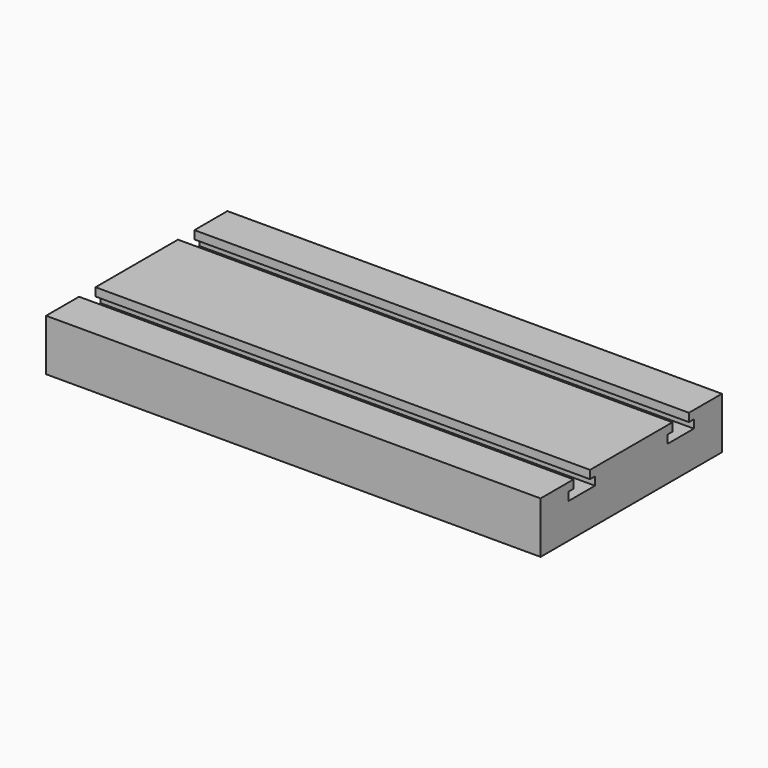
from build123d import *

# Parameters (mm, degrees)
F0_W          = 69.85
F0_H          = 15.875
F1_DEPTH      = 76.2
F1_DEPTH_BACK = 76.2
F3_DEPTH      = 76.201
F3_DEPTH_BACK = 76.201


# Not quite as in the source:
# - a pattern or mirror of a feature is missing from the dataset's text; its kind, count and spacing are read off the source's solid


with BuildPart() as f1:
    # F0 (on Right) → F1 (new body, two sides)
    with BuildSketch(Plane.YZ) as f1_sk:
        with Locations((0, -31.75)):
            Rectangle(F0_W, F0_H)
    extrude(amount=F1_DEPTH)
    extrude(f1_sk.sketch, amount=-F1_DEPTH_BACK)

    # F2 (on Right) → F3 (cut, two sides)
    with BuildSketch(Plane.YZ) as f3_sk:
        Polygon((-15.875, -26.3525), (-15.875, -23.8125), (-22.225, -23.8125), (-22.225, -26.3525), (-24.13, -26.3525), (-24.13, -28.8925), (-13.97, -28.8925), (-13.97, -26.3525), align=None)
    f3 = extrude(amount=-F3_DEPTH, mode=Mode.SUBTRACT) + extrude(f3_sk.sketch, amount=F3_DEPTH_BACK, mode=Mode.SUBTRACT)

    # F3_copies: F3 across plane
    add(f3.mirror(Plane.ZX), mode=Mode.SUBTRACT)


solid = f1.part
